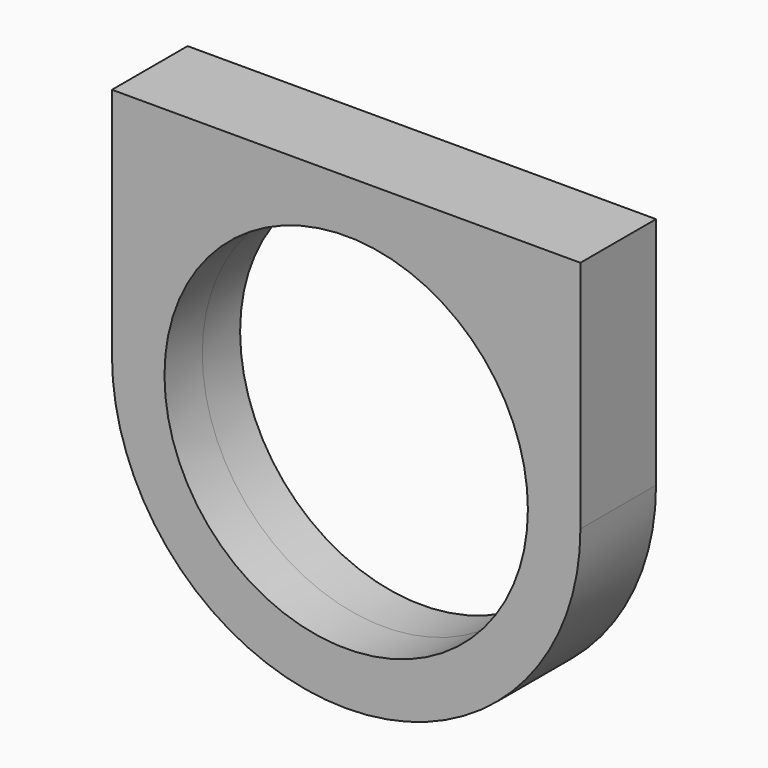
from build123d import *

# Parameters (mm, degrees)
F0_R          = 8.65
F1_DEPTH      = 2.25
F1_DEPTH_BACK = 2.25


# Not quite as in the source:
# - the program builds the solid bodies; features that only make, move or delete a surface that nothing else refers to are left out


with BuildPart() as f1:
    # F0 (on Front) → F1 (new body, two sides)
    with BuildSketch(Plane.XZ) as f1_sk:
        with BuildLine():
            ThreePointArc((-11.15, 0), (0, -11.15), (11.15, 0))
            ThreePointArc((11.15, 0), (7.8842406102, 7.8842406102), (0, 11.15))
            ThreePointArc((0, 11.15), (-7.8842406102, 7.8842406102), (-11.15, 0))
        make_face()
        Circle(F0_R, mode=Mode.SUBTRACT)
        with BuildLine():
            ThreePointArc((-11.15, 0), (-7.8842406102, 7.8842406102), (0, 11.15))
            Line((0, 11.15), (-4, 11.15))
            Line((-4, 11.15), (-9.15, 11.15))
            Line((-9.15, 11.15), (-11.15, 11.15))
            Line((-11.15, 11.15), (-11.15, 0))
        make_face()
        with BuildLine():
            ThreePointArc((0, 11.15), (7.8842406102, 7.8842406102), (11.15, 0))
            Line((11.15, 0), (11.15, 11.15))
            Line((11.15, 11.15), (0, 11.15))
        make_face()
    extrude(amount=F1_DEPTH)
    extrude(f1_sk.sketch, amount=-F1_DEPTH_BACK)


solid = f1.part
